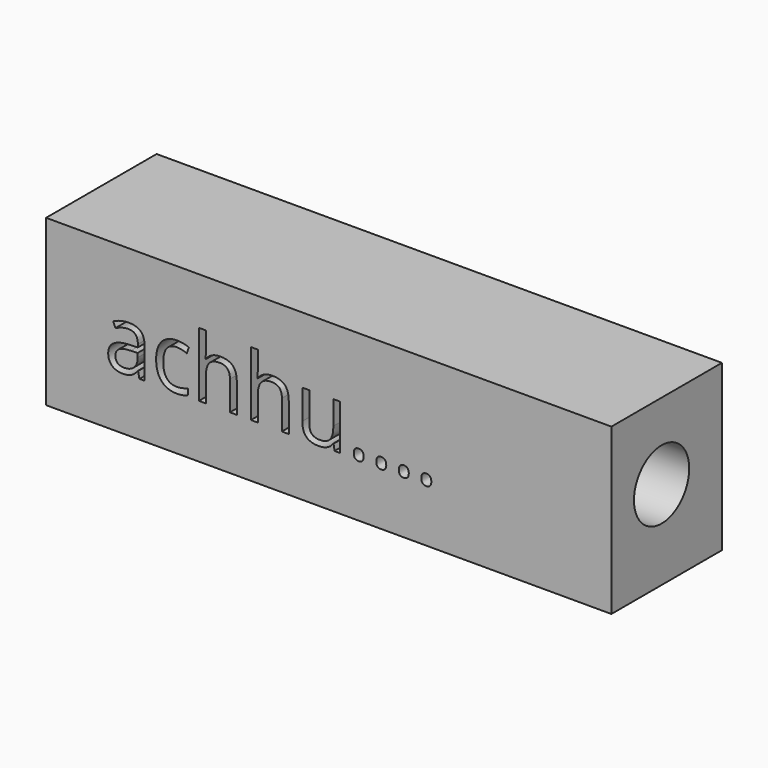
from build123d import *

# Parameters (mm, degrees)
F0_W         = 174.0783005953
F0_H         = 42.5428263843
F1_DEPTH     = 50.8
F2_R         = 10.6286214809
F3_DEPTH     = 177.8
F4_TEXT_SIZE = 26.0599656031
F5_DEPTH     = 50.8


# Not quite as in the source:
# - Text() gives the source's letters only with a copy of the font that has no kerning and outlines rounded to 1/6400 em; it was checked with that copy


with BuildPart() as f1:
    # F0 (on Top) → F1 (new body)
    with BuildSketch(Plane.XY):
        with Locations((24.0931287408, 1.9534900784)):
            Rectangle(F0_W, F0_H)
    extrude(amount=F1_DEPTH)

    # F2 (on face) → F3 (cut)
    with BuildSketch(Plane(origin=(-62.9460215569, 0, 0), x_dir=(0, -1, 0), z_dir=(-1, 0, 0))):
        with Locations((0, 27.2791553289)):
            Circle(F2_R)
    extrude(amount=-F3_DEPTH, mode=Mode.SUBTRACT)

    # F4 (on face) → F5 (cut)
    with BuildSketch(Plane.XZ.offset(19.3179231137)):
        with Locations((-45.0102798641, 16.4760556072)):
            Text('achhu....', F4_TEXT_SIZE, font='Open Sans', text_align=(TextAlign.LEFT, TextAlign.BOTTOM))
    extrude(amount=-F5_DEPTH, mode=Mode.SUBTRACT)


solid = f1.part
